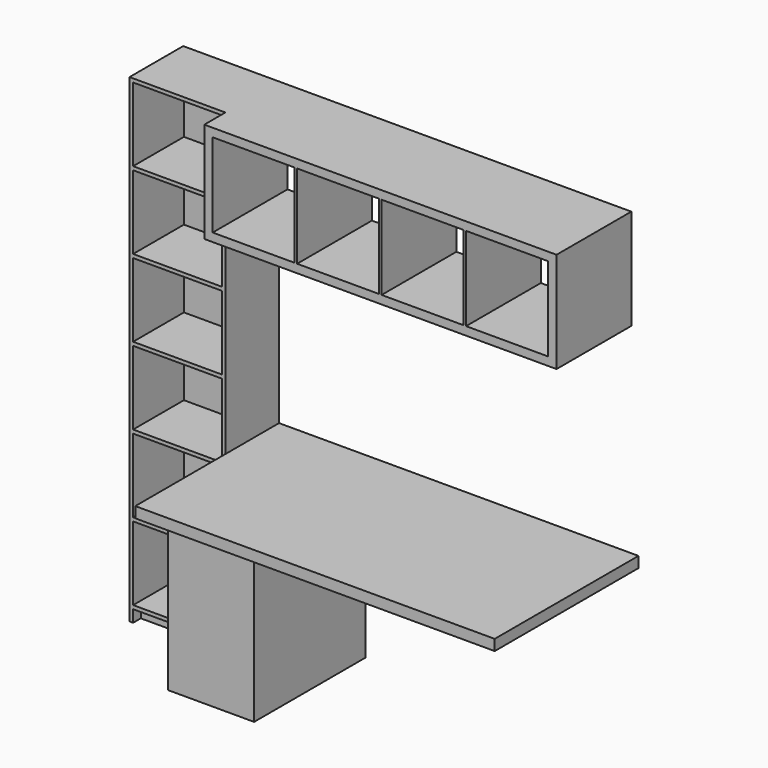
from build123d import *

# Parameters (mm, degrees)
F0_W      = 1500
F0_H      = 750
F1_DEPTH  = 45
F2_W      = 360
F2_H      = 580
F3_DEPTH  = 700
F8_W      = 280
F8_H      = 2000
F9_DEPTH  = 400
F10_W     = 370
F10_H     = 307.5
F11_DEPTH = 265
F10_H_2   = 50
F12_DEPTH = 40
F13_W     = 110
F13_H     = 420
F13_W_2   = 280
F14_DEPTH = 1470
F15_W     = 342.5
F15_H     = 350
F16_DEPTH = 390


# Not quite as in the source:
# - the program builds the solid bodies; features that only make, move or delete a surface that nothing else refers to are left out


with BuildPart() as f1:
    # F0 (on Top) → F1 (new body)
    with BuildSketch(Plane.XY):
        with Locations((19.0651228034, -0.7792990655)):
            Rectangle(F0_W, F0_H)
    extrude(amount=F1_DEPTH)


with BuildPart() as f3:
    # F2 (on face) → F3 (new body)
    with BuildSketch(Plane(origin=(0, 0, 0), x_dir=(1, 0, 0), z_dir=(0, 0, -1))):
        with Locations((-550.9348771966, -84.2207009345)):
            Rectangle(F2_W, F2_H)
    extrude(amount=F3_DEPTH)


with BuildPart() as f9:
    # F8 (on face) → F9 (new body)
    with BuildSketch(Plane(origin=(-730.9348771966, 0, 0), x_dir=(0, -1, 0), z_dir=(-1, 0, 0))):
        with Locations((-234.2207009345, 300)):
            Rectangle(F8_W, F8_H)
    extrude(amount=F9_DEPTH)

    # F10 (on face) → F11 (cut)
    with BuildSketch(Plane.XZ.offset(-94.2207009345)):
        with Locations((-930.9348771966, -481.25)):
            Rectangle(F10_W, F10_H)
        with Locations((-930.9348771966, -158.75)):
            Rectangle(F10_W, F10_H)
        with Locations((-930.9348771966, 163.75)):
            Rectangle(F10_W, F10_H)
        with Locations((-930.9348771966, 486.25)):
            Rectangle(F10_W, F10_H)
        with Locations((-930.9348771966, 808.75)):
            Rectangle(F10_W, F10_H)
        with Locations((-930.9348771966, 1131.25)):
            Rectangle(F10_W, F10_H)
    extrude(amount=-F11_DEPTH, mode=Mode.SUBTRACT)

    # F10 (on face) → F12 (cut)
    with BuildSketch(Plane.XZ.offset(-94.2207009345)):
        with Locations((-930.9348771966, -675)):
            Rectangle(F10_W, F10_H_2)
    extrude(amount=-F12_DEPTH, mode=Mode.SUBTRACT)

    # F13 (on face) → F14 (join)
    with BuildSketch(Plane.YZ.offset(-730.9348771966)):
        with Locations((39.2207009345, 1090)):
            Rectangle(F13_W, F13_H)
        with Locations((234.2207009345, 1090)):
            Rectangle(F13_W_2, F13_H)
    extrude(amount=F14_DEPTH)

    # F15 (on face) → F16 (cut)
    with BuildSketch(Plane.XZ.offset(15.7792990655)):
        with Locations((-524.6848771966, 1090)):
            Rectangle(F15_W, F15_H)
        with Locations((-172.1848771966, 1090)):
            Rectangle(F15_W, F15_H)
        with Locations((180.3151228034, 1090)):
            Rectangle(F15_W, F15_H)
        with Locations((532.8151228034, 1090)):
            Rectangle(F15_W, F15_H)
    extrude(amount=-F16_DEPTH, mode=Mode.SUBTRACT)


solid = Compound([f1.part, f3.part, f9.part])
